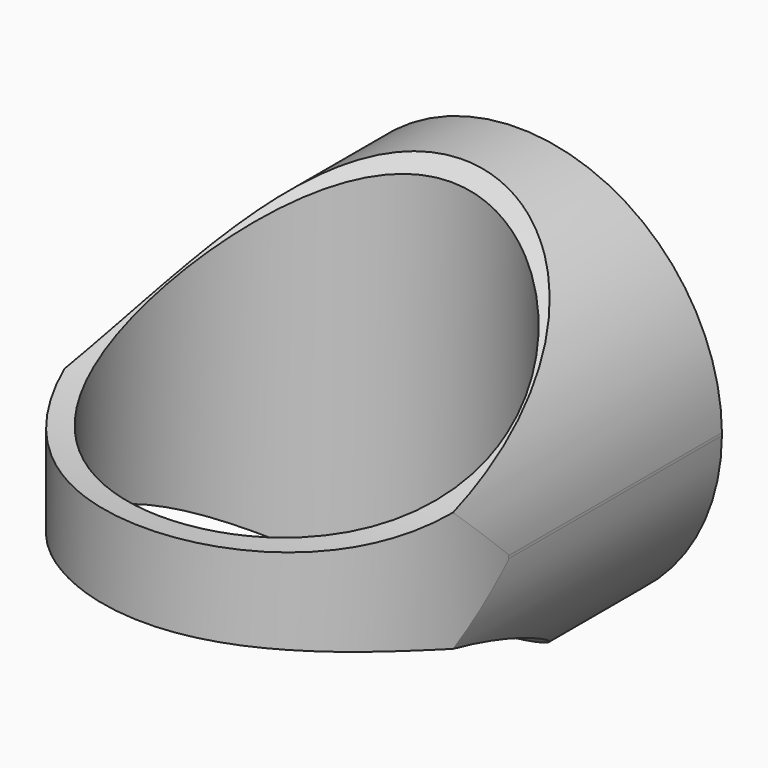
from build123d import *

# Parameters (mm, degrees)
F2_DEPTH     = 14.6
F3_R         = 25
F3_R_2       = 7.3
F4_DEPTH     = 25
F5_R         = 20.6
F6_DEPTH     = 59.1926729486
F7_TEXT_SIZE = 12.9944867998
F8_DEPTH     = 0.5


# Not quite as in the source:
# - Text() gives the source's letters only with a copy of the font that has no kerning and outlines rounded to 1/6400 em; it was checked with that copy


with BuildPart() as f2:
    # F1 (on Top) → F2 (new body)
    with BuildSketch(Plane.XY):
        with BuildLine():
            ThreePointArc((-58.391477238, -6.6704245953), (-51.9256807666, -0.1028117628), (-45.3918298185, -6.6027236171))
            ThreePointArc((-45.3918298185, -6.6027236171), (-45.3919179642, -6.6365745652), (-45.392182399, -6.6704245953))
            Line((-45.392182399, -6.6704245953), (-44.5921437583, -6.6704245953))
            ThreePointArc((-44.5921437583, -6.6704245953), (-44.5919083039, -6.6365744701), (-44.5918298185, -6.6027236171))
            Line((-44.5918298185, -6.6027236171), (-44.5918298185, 2.8972763829))
            Line((-44.5918298185, 2.8972763829), (-59.1915158787, 2.8972763829))
            Line((-59.1915158787, 2.8972763829), (-59.1915158787, -6.5350226389))
            Line((-59.1915158787, -6.5350226389), (-59.1915158787, -6.6704245953))
            Line((-59.1915158787, -6.6704245953), (-58.391477238, -6.6704245953))
        make_face()
        with BuildLine():
            ThreePointArc((-45.392182399, -6.6704245953), (-51.8918298185, -13.1027236171), (-58.391477238, -6.6704245953))
            Line((-58.391477238, -6.6704245953), (-59.1915158787, -6.6704245953))
            ThreePointArc((-59.1915158787, -6.6704245953), (-51.8918298185, -13.9027236171), (-44.5921437583, -6.6704245953))
            Line((-44.5921437583, -6.6704245953), (-45.392182399, -6.6704245953))
        make_face()
        with BuildLine():
            ThreePointArc((-59.1915158787, -6.5350226389), (-59.1918298185, -6.6027236171), (-59.1915158787, -6.6704245953))
            Line((-59.1915158787, -6.6704245953), (-59.1915158787, -6.5350226389))
        make_face()
        with BuildLine():
            ThreePointArc((-44.5918298185, -6.6027236171), (-44.5919083039, -6.6365744701), (-44.5921437583, -6.6704245953))
            Line((-44.5921437583, -6.6704245953), (-44.5918298185, -6.6704245953))
            Line((-44.5918298185, -6.6704245953), (-44.5918298185, -6.6027236171))
        make_face()
    extrude(amount=F2_DEPTH)

    # F3 (on face) → F4 (cut)
    with BuildSketch(Plane(origin=(0, 2.8972763829, 0), x_dir=(-1, 0, 0), z_dir=(0, 1, 0))):
        with Locations((51.8916728486, 7.3)):
            Circle(F3_R)
        with Locations((51.8916728486, 7.3)):
            Circle(F3_R_2, mode=Mode.SUBTRACT)
    extrude(amount=-F4_DEPTH, mode=Mode.SUBTRACT)

    # F5 (on Right) → F6 (cut, through all)
    with BuildSketch(Plane.YZ):
        with Locations((-13.9027236171, 29.4)):
            Circle(F5_R)
        with Locations((-13.9027236171, -14.8)):
            Circle(F5_R)
    extrude(amount=-F6_DEPTH, mode=Mode.SUBTRACT)

    # F7 (on face) → F8 (cut)
    with BuildSketch(Plane(origin=(0, 2.8972763829, 0), x_dir=(-1, 0, 0), z_dir=(0, 1, 0))):
        with Locations((48.7295202911, 3.2826147508)):
            Text('L', F7_TEXT_SIZE, font='Open Sans', text_align=(TextAlign.LEFT, TextAlign.BOTTOM))
    extrude(amount=-F8_DEPTH, mode=Mode.SUBTRACT)


solid = f2.part
